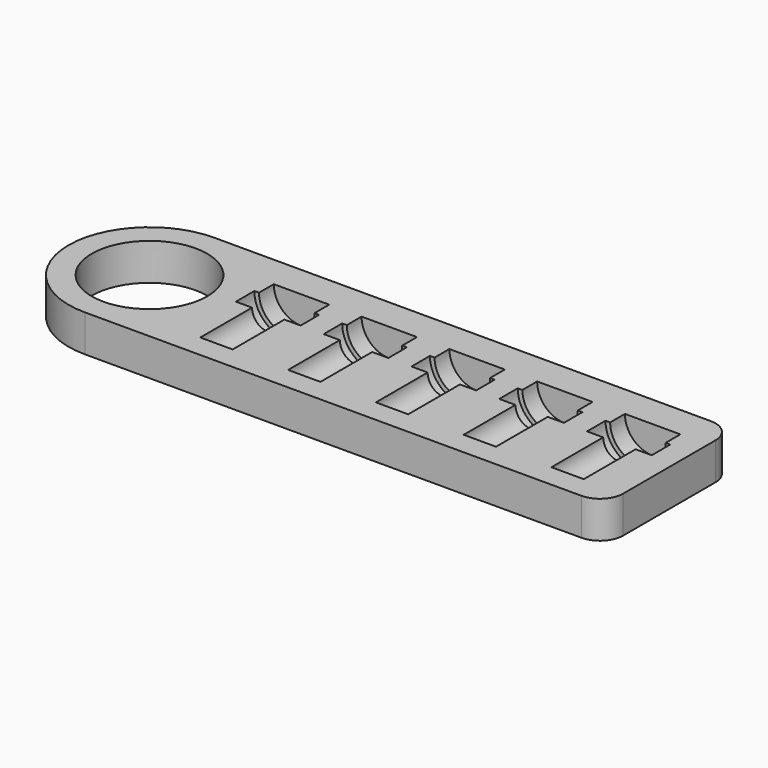
from build123d import *

# Parameters (mm, degrees)
F0_R         = 12.5
F1_DEPTH     = 8
F8_TEXT_SIZE = 5.5555555556
F9_DEPTH     = 1


# Not quite as in the source:
# - Text() gives the source's letters only with a copy of the font that has no kerning and outlines rounded to 1/6400 em; it was checked with that copy


with BuildPart() as f1:
    # F0 (on Top) → F1 (new body)
    with BuildSketch(Plane.XY):
        with BuildLine():
            ThreePointArc((0, 17.5), (5.1256313292, 5.1256313292), (17.5, 0))
            Line((17.5, 0), (125, 0))
            ThreePointArc((125, 0), (128.5355339059, 1.4644660941), (130, 5))
            Line((130, 5), (130, 30))
            ThreePointArc((130, 30), (128.5355339059, 33.5355339059), (125, 35))
            Line((125, 35), (17.5, 35))
            ThreePointArc((17.5, 35), (5.1256313292, 29.8743686708), (0, 17.5))
        make_face()
        with Locations((17.5, 17.5)):
            Circle(F0_R, mode=Mode.SUBTRACT)
    extrude(amount=F1_DEPTH)

    # F2 (on face) → F3 (revolve, cut)
    with BuildSketch(Plane.XY.offset(8)):
        Polygon((42, 19), (42, 5), (45.5, 5), (45.5, 19), (49, 19), (49, 24), (48, 24), (48, 28), (42, 28), (42, 24), align=None)
    revolve(axis=Axis((42, 21.5, 8), (0, 1, 0)), mode=Mode.SUBTRACT)

    # F2 (on face) → F4 (revolve, cut)
    with BuildSketch(Plane.XY.offset(8)):
        Polygon((61, 19), (61, 5), (64.5, 5), (64.5, 19), (68, 19), (68, 24), (67, 24), (67, 28), (61, 28), (61, 24), align=None)
    revolve(axis=Axis((61, 21.5, 8), (0, 1, 0)), mode=Mode.SUBTRACT)

    # F2 (on face) → F5 (revolve, cut)
    with BuildSketch(Plane.XY.offset(8)):
        Polygon((80, 19), (80, 5), (83.5, 5), (83.5, 19), (87, 19), (87, 24), (86, 24), (86, 28), (80, 28), (80, 24), align=None)
    revolve(axis=Axis((80, 12, 8), (0, 1, 0)), mode=Mode.SUBTRACT)

    # F2 (on face) → F6 (revolve, cut)
    with BuildSketch(Plane.XY.offset(8)):
        Polygon((99, 19), (99, 5), (102.5, 5), (102.5, 19), (106, 19), (106, 24), (105, 24), (105, 28), (99, 28), (99, 24), align=None)
    revolve(axis=Axis((99, 12, 8), (0, 1, 0)), mode=Mode.SUBTRACT)

    # F2 (on face) → F7 (revolve, cut)
    with BuildSketch(Plane.XY.offset(8)):
        Polygon((118, 19), (118, 5), (121.5, 5), (121.5, 19), (125, 19), (125, 24), (124, 24), (124, 28), (118, 28), (118, 24), align=None)
    revolve(axis=Axis((118, 12, 8), (0, 1, 0)), mode=Mode.SUBTRACT)

    # F8 (on face) → F9 (cut)
    with BuildSketch(Plane(origin=(0, 0, 0), x_dir=(1, 0, 0), z_dir=(0, 0, -1))):
        with Locations((30, -9)):
            Text('869', F8_TEXT_SIZE, font='Open Sans', text_align=(TextAlign.LEFT, TextAlign.BOTTOM))
    extrude(amount=-F9_DEPTH, mode=Mode.SUBTRACT)


solid = f1.part
